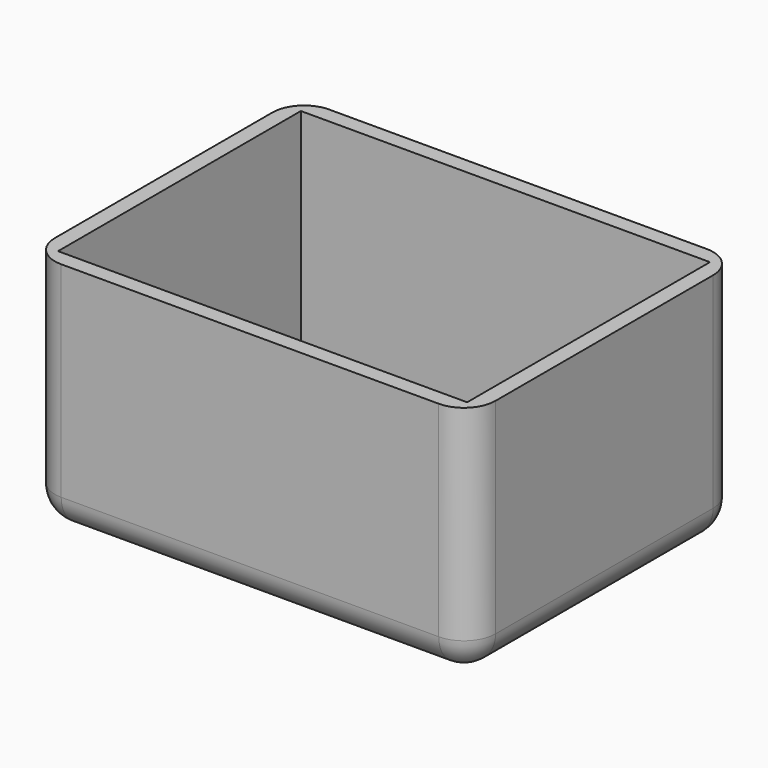
from build123d import *

# Parameters (mm, degrees)
F0_W         = 70.9387809038
F0_H         = 53.9411939681
F1_DEPTH     = 38.1
F2_T         = -2.54
F3_R         = 5.08
F4_T1_DEPTH  = 43.7811939681
F4_T3_DEPTH  = 45.72
F4_S7_W      = 5.08
F4_S7_H      = 5.08
F4_T8_DEPTH  = 5.08
F4_S13_W     = 5.08
F4_S13_H     = 5.08
F4_T14_DEPTH = 5.08
F4_T18_ANGLE = 90
F4_T20_ANGLE = 90


# Not quite as in the source:
# - a fillet or chamfer that OpenCascade refuses, or shapes differently, is made with other operations: its cross-section is extruded or revolved along the edge and cut away or added


with BuildPart() as f1:
    # F0 (on Top) → F1 (new body)
    with BuildSketch(Plane.XY):
        Rectangle(F0_W, F0_H)
    extrude(amount=F1_DEPTH)

    # F2
    f2_openings = [f1.faces().sort_by_distance(p)[0] for p in [
        (0, 0, 38.1),
    ]]
    offset(amount=F2_T, openings=f2_openings)

    # F3
    f3_edges = [f1.edges().sort_by_distance(p)[0] for p in [
        (0, 26.970597, 0),
        (0, -26.970597, 0),
        (-35.46939, 26.970597, 19.05),
        (35.46939, -26.970597, 19.05),
    ]]
    fillet(f3_edges, radius=F3_R)

    # F4: fillet of radius 5.08 on 3 edges, made by hand

    # F4_s2 → F4_t1 (cut)
    with BuildSketch(Plane.XZ.offset(-21.890596984)):
        with BuildLine():
            ThreePointArc((30.3893904519, 0), (33.9814929003, 1.4878975516), (35.4693904519, 5.08))
            Line((35.4693904519, 5.08), (35.4693904519, 0))
            Line((35.4693904519, 0), (30.3893904519, 0))
        make_face()
        with BuildLine():
            ThreePointArc((-35.4693904519, 5.08), (-33.9814929003, 1.4878975516), (-30.3893904519, 0))
            Line((-30.3893904519, 0), (-35.4693904519, 0))
            Line((-35.4693904519, 0), (-35.4693904519, 5.08))
        make_face()
    extrude(amount=F4_T1_DEPTH, mode=Mode.SUBTRACT)

    # F4_s4 → F4_t3 (cut)
    with BuildSketch(Plane.XY.offset(5.08)):
        with BuildLine():
            ThreePointArc((-30.3893904519, -26.970596984), (-33.9814929003, -25.4826994325), (-35.4693904519, -21.890596984))
            Line((-35.4693904519, -21.890596984), (-35.4693904519, -26.970596984))
            Line((-35.4693904519, -26.970596984), (-30.3893904519, -26.970596984))
        make_face()
        with BuildLine():
            ThreePointArc((35.4693904519, 21.890596984), (33.9814929003, 25.4826994325), (30.3893904519, 26.970596984))
            Line((30.3893904519, 26.970596984), (35.4693904519, 26.970596984))
            Line((35.4693904519, 26.970596984), (35.4693904519, 21.890596984))
        make_face()
    extrude(amount=F4_T3_DEPTH, mode=Mode.SUBTRACT)


with BuildPart() as f4_tool6:
    # F4_s7 → F4_t8 (new body)
    with BuildSketch(Plane.YZ.offset(-30.3893904519)):
        with Locations((24.430596984, 2.54)):
            Rectangle(F4_S7_W, F4_S7_H)
    extrude(amount=-F4_T8_DEPTH)

    # F4_s9 → F4_t10 (revolve, cut)
    with BuildSketch(Plane(origin=(-30.3893904519, 21.890596984, 5.08), x_dir=(0, -0.7071067812, 0.7071067812), z_dir=(0, -0.7071067812, -0.7071067812))):
        with BuildLine():
            ThreePointArc((0, -5.08), (5.08, 0), (0, 5.08))
            Line((0, 5.08), (0, -5.08))
        make_face()
    revolve(axis=Axis((-30.3893904519, 21.890596984, 5.08), (-1, 0, 0)), mode=Mode.SUBTRACT)


with BuildPart() as f1_1:
    add(f1.part)

    # F4_t5: cut F4_tool6
    add(f4_tool6.part, mode=Mode.SUBTRACT)


with BuildPart() as f4_tool12:
    # F4_s13 → F4_t14 (new body)
    with BuildSketch(Plane.XY.offset(5.08)):
        with Locations((32.9293904519, -24.430596984)):
            Rectangle(F4_S13_W, F4_S13_H)
    extrude(amount=-F4_T14_DEPTH)

    # F4_s15 → F4_t16 (revolve, cut)
    with BuildSketch(Plane(origin=(30.3893904519, -21.890596984, 5.08), x_dir=(-0.7071067812, 0.7071067812, 0), z_dir=(-0.7071067812, -0.7071067812, 0))):
        with BuildLine():
            ThreePointArc((0, -5.08), (5.08, 0), (0, 5.08))
            Line((0, 5.08), (0, -5.08))
        make_face()
    revolve(axis=Axis((30.3893904519, -21.890596984, 5.08), (0, 0, -1)), mode=Mode.SUBTRACT)


with BuildPart() as f1_2:
    add(f1_1.part)

    # F4_t11: cut F4_tool12
    add(f4_tool12.part, mode=Mode.SUBTRACT)

    # F4_s17 → F4_t18 (revolve, cut)
    with BuildSketch(Plane.XY.offset(5.08)):
        with BuildLine():
            ThreePointArc((-35.4693904519, -21.890596984), (-33.9814929003, -25.4826994325), (-30.3893904519, -26.970596984))
            Line((-30.3893904519, -26.970596984), (-35.4693904519, -26.970596984))
            Line((-35.4693904519, -26.970596984), (-35.4693904519, -21.890596984))
        make_face()
    revolve(axis=Axis((-35.4693904519, -21.890596984, 5.08), (1, 0, 0)), revolution_arc=F4_T18_ANGLE, mode=Mode.SUBTRACT)

    # F4_s19 → F4_t20 (revolve, cut)
    with BuildSketch(Plane.XY.offset(5.08)):
        with BuildLine():
            ThreePointArc((35.4693904519, 21.890596984), (33.9814929003, 25.4826994325), (30.3893904519, 26.970596984))
            Line((30.3893904519, 26.970596984), (35.4693904519, 26.970596984))
            Line((35.4693904519, 26.970596984), (35.4693904519, 21.890596984))
        make_face()
    revolve(axis=Axis((35.4693904519, 21.890596984, 5.08), (-1, 0, 0)), revolution_arc=F4_T20_ANGLE, mode=Mode.SUBTRACT)


solid = f1_2.part
